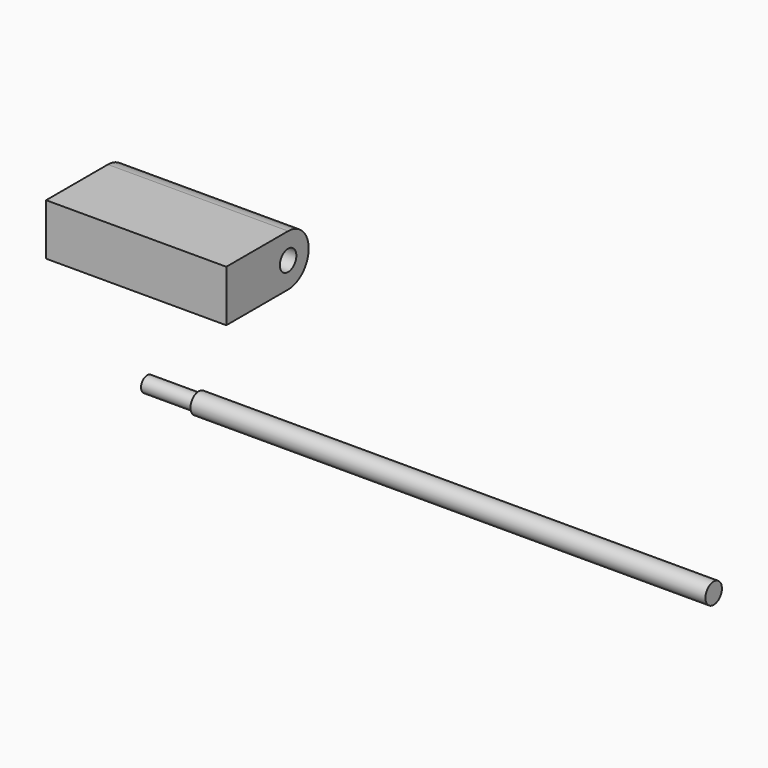
from build123d import *

# Parameters (mm, degrees)
F0_R      = 3
F1_DEPTH  = 20
F0_R_2    = 4
F1_FACE_R = 3
F2_DEPTH  = 200
F3_W      = 70
F3_H      = 40
F4_DEPTH  = 20
F5_R      = 9.99999
F6_R      = 4
F7_DEPTH  = 70.001


# Not quite as in the source:
# - a fillet or chamfer is up to 0.001 mm smaller than in the source, because OpenCascade refuses the exact size


with BuildPart() as f1:
    # F0 (on Right) → F1 (new body)
    with BuildSketch(Plane.YZ):
        with Locations((-69.3261250854, 0)):
            Circle(F0_R)
    extrude(amount=-F1_DEPTH)

    # F0 (on Right) + F1_face (on face) → F2 (join)
    with BuildSketch(Plane.YZ):
        with Locations((-69.3261250854, 0)):
            Circle(F0_R_2)
        with Locations((-69.3261250854, 0)):
            Circle(F0_R, mode=Mode.SUBTRACT)
    with BuildSketch(Plane(origin=(0, -69.3261250854, 0), x_dir=(0, 1, 0), z_dir=(1, 0, 0))):
        Circle(F1_FACE_R)
    extrude(amount=F2_DEPTH)


with BuildPart() as f4:
    # F3 (on Top) → F4 (new body)
    with BuildSketch(Plane.XY):
        with Locations((-60.3385819857, -4.25943546)):
            Rectangle(F3_W, F3_H)
    extrude(amount=F4_DEPTH)

    # F5 (radius 10 in the source; OpenCascade refuses exactly that, so slightly less here)
    f5_edges = [f4.edges().sort_by_distance(p)[0] for p in [
        (-60.338582, 15.740565, 20),
        (-60.338582, 15.740565, 0),
    ]]
    fillet(f5_edges, radius=F5_R)

    # F6 (on face) → F7 (cut, through all)
    with BuildSketch(Plane.YZ.offset(-25.3385819857)):
        with Locations((5.74056454, 10)):
            Circle(F6_R)
    extrude(amount=-F7_DEPTH, mode=Mode.SUBTRACT)


solid = Compound([f1.part, f4.part])
